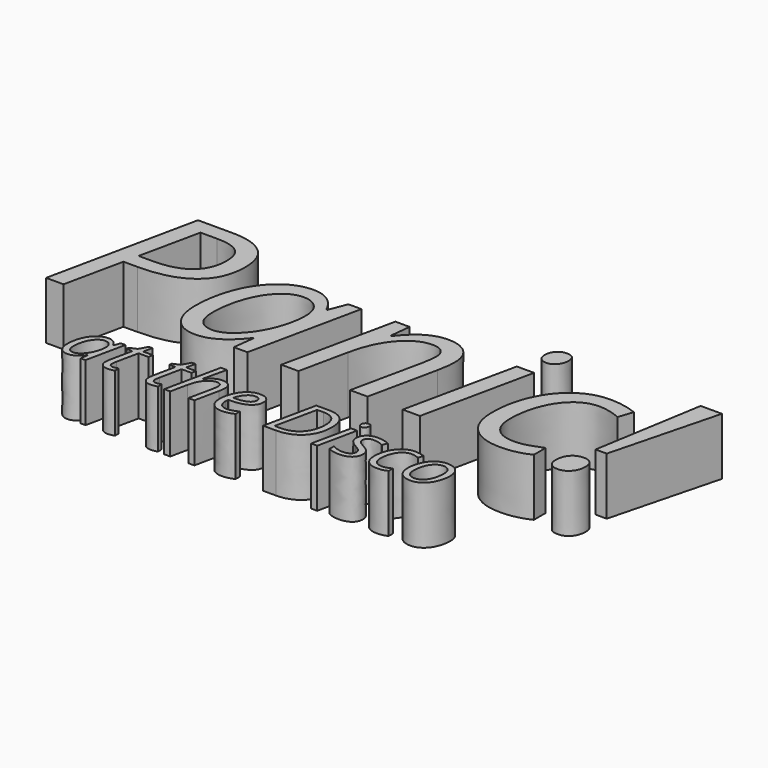
from build123d import *

# Parameters (mm, degrees)
F0_TEXT_SIZE   = 18.645134858
F0_TEXT_SIZE_2 = 6.5257973296
F1_DEPTH       = 5.08


# Not quite as in the source:
# - Text() gives the source's letters only with a copy of the font that has no kerning and outlines rounded to 1/6400 em; it was checked with that copy


with BuildPart() as f1:
    # F0 (on Top) → F1 (new body)
    with BuildSketch(Plane.XY):
        with Locations((-62.1394165792, 7.9204514623)):
            Text('Panic!', F0_TEXT_SIZE, font='Open Sans', font_style=FontStyle.ITALIC, text_align=(TextAlign.LEFT, TextAlign.BOTTOM))
        with Locations((-54.3532110751, 0)):
            Text('at the Disco', F0_TEXT_SIZE_2, font='Open Sans', font_style=FontStyle.ITALIC, text_align=(TextAlign.LEFT, TextAlign.BOTTOM))
    extrude(amount=F1_DEPTH)


solid = f1.part
